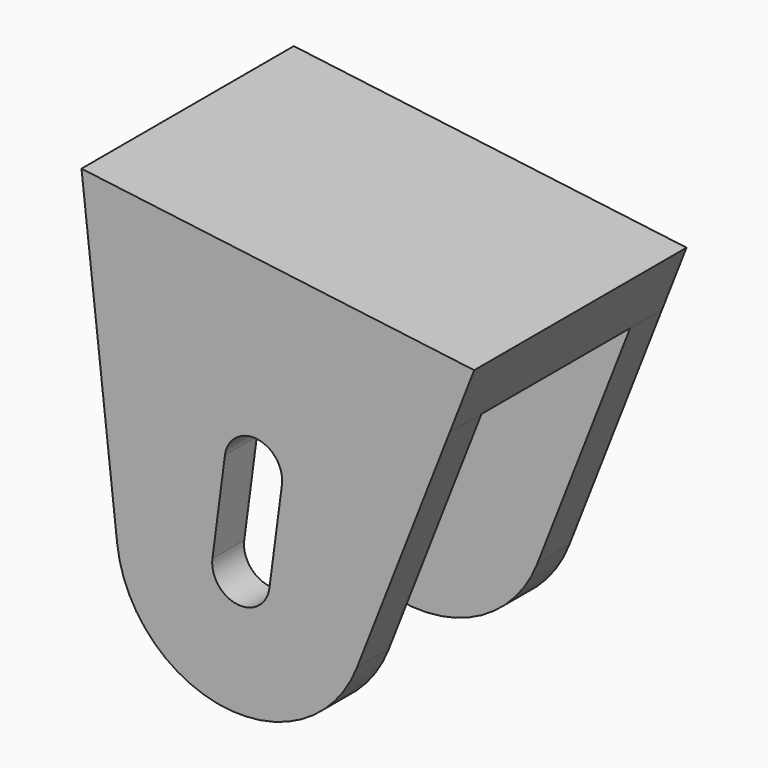
from build123d import *

# Parameters (mm, degrees)
F1_DEPTH = 7.5
F2_DEPTH = 5.25


# Not quite as in the source:
# - ends of sketch curves that miss each other by under 0.0002 mm in the source are joined


with BuildPart() as f1:
    # F0 (on Front) → F1 (new body, symmetric)
    with BuildSketch(Plane.XZ):
        with BuildLine():
            ThreePointArc((-11.0043239024, 7.1529938994), (-0.6435162461, 7.0398408721), (9.3939724206, 4.4692455787))
            Line((9.3939724206, 4.4692455787), (10.7793952497, 8.0129774852))
            Line((10.7793952497, 8.0129774852), (-11.4156674583, 10.8236569963))
            Line((-11.4156674583, 10.8236569963), (-11.0043239024, 7.1529938994))
        make_face()
        with BuildLine():
            Line((4.1502654463, -8.9435067945), (9.39397455, 4.4692447462))
            ThreePointArc((9.39397455, 4.4692447462), (-0.6435162461, 7.0398408721), (-11.0043239024, 7.1529938994))
            Line((-11.0043239024, 7.1529938994), (-9.3998677417, -7.1645337772))
            ThreePointArc((-9.3998677417, -7.1645337772), (-3.3213281789, -13.3593367926), (4.1502654463, -8.9435067945))
        make_face()
        with BuildLine():
            ThreePointArc((-3.3084953622, -0.8006877888), (-1.4860286023, 0.5975869129), (-0.0877539006, -1.2248798469))
            Line((-0.0877539006, -1.2248798469), (-0.7947424255, -6.5927825509))
            ThreePointArc((-0.7947424255, -6.5927825509), (-2.6172092627, -7.9910572424), (-4.0154839644, -6.1685904826))
            Line((-4.0154839644, -6.1685904826), (-3.3084953622, -0.8006877888))
        make_face(mode=Mode.SUBTRACT)
    extrude(amount=F1_DEPTH, both=True)

    # F0 (on Front) → F2 (cut, symmetric)
    with BuildSketch(Plane.XZ):
        with BuildLine():
            Line((4.1502654463, -8.9435067945), (9.39397455, 4.4692447462))
            ThreePointArc((9.39397455, 4.4692447462), (-0.6435162461, 7.0398408721), (-11.0043239024, 7.1529938994))
            Line((-11.0043239024, 7.1529938994), (-9.3998677417, -7.1645337772))
            ThreePointArc((-9.3998677417, -7.1645337772), (-3.3213281789, -13.3593367926), (4.1502654463, -8.9435067945))
        make_face()
        with BuildLine():
            ThreePointArc((-3.3084953622, -0.8006877888), (-1.4860286023, 0.5975869129), (-0.0877539006, -1.2248798469))
            Line((-0.0877539006, -1.2248798469), (-0.7947424255, -6.5927825509))
            ThreePointArc((-0.7947424255, -6.5927825509), (-2.6172092627, -7.9910572424), (-4.0154839644, -6.1685904826))
            Line((-4.0154839644, -6.1685904826), (-3.3084953622, -0.8006877888))
        make_face(mode=Mode.SUBTRACT)
    extrude(amount=F2_DEPTH, both=True, mode=Mode.SUBTRACT)


solid = f1.part
